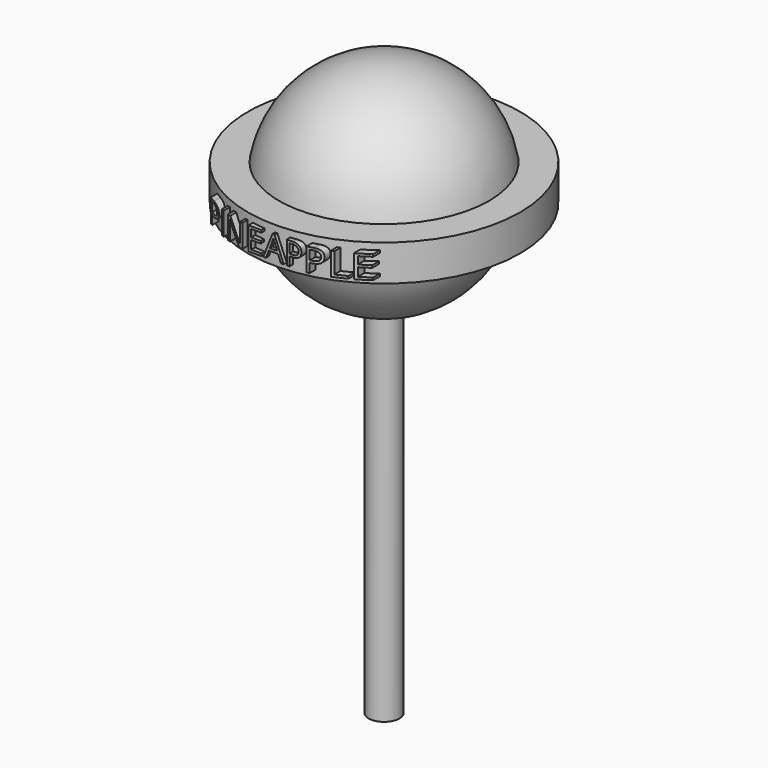
from build123d import *

# Parameters (mm, degrees)
F0_W         = 0.8679474239
F0_H         = 7.7723114803
F0_W_2       = 7.6306914445
F2_TEXT_SIZE = 6.9138606907
F3_DEPTH     = 30


# Not quite as in the source:
# - Text() gives the source's letters only with a copy of the font that has no kerning and outlines rounded to 1/6400 em; it was checked with that copy


with BuildPart() as f1:
    # F0 (on Front) → F1 (revolve)
    with BuildSketch(Plane.XZ):
        with BuildLine():
            Line((0, -18.649796024), (0, -22.9185808741))
            ThreePointArc((0, -22.9185808741), (1.6568504998, -22.8586131623), (3.305030521, -22.6790238445))
            Line((3.305030521, -22.6790238445), (3.305030521, -18.649796024))
            Line((3.305030521, -18.649796024), (0, -18.649796024))
        make_face()
        with BuildLine():
            ThreePointArc((3.305030521, -22.6790238445), (1.6568504998, -22.8586131623), (0, -22.9185808741))
            Line((0, -22.9185808741), (0, -100.3312021494))
            Line((0, -100.3312021494), (3.305030521, -100.3312021494))
            Line((3.305030521, -100.3312021494), (3.305030521, -22.6790238445))
        make_face()
        with BuildLine():
            Line((3.305030521, -18.649796024), (3.305030521, -22.6790238445))
            ThreePointArc((3.305030521, -22.6790238445), (15.9965132556, -16.4125839814), (22.5867027883, -3.8861557401))
            Line((22.5867027883, -3.8861557401), (0, -3.8861557401))
            Line((0, -3.8861557401), (0, -18.649796024))
            Line((0, -18.649796024), (3.305030521, -18.649796024))
        make_face()
        with BuildLine():
            Line((0, -3.8861557401), (22.5867027883, -3.8861557401))
            ThreePointArc((22.5867027883, -3.8861557401), (22.9185808741, 0), (22.5867027883, 3.8861557401))
            Line((22.5867027883, 3.8861557401), (0, 3.8861557401))
            Line((0, 3.8861557401), (0, -3.8861557401))
        make_face()
        with BuildLine():
            ThreePointArc((22.5867027883, 3.8861557401), (22.9185808741, 0), (22.5867027883, -3.8861557401))
            Line((22.5867027883, -3.8861557401), (29.2731001973, -3.8861557401))
            Line((29.2731001973, -3.8861557401), (29.2731001973, 3.8861557401))
            Line((29.2731001973, 3.8861557401), (22.5867027883, 3.8861557401))
        make_face()
        with Locations((-0.4339737119, 0)):
            Rectangle(F0_W, F0_H)
        with BuildLine():
            Line((0, 3.8861557401), (22.5867027883, 3.8861557401))
            ThreePointArc((22.5867027883, 3.8861557401), (14.7681443429, 17.5260737746), (0, 22.9185808741))
            Line((0, 22.9185808741), (0, 3.8861557401))
        make_face()
        with Locations((-4.6832931461, 0)):
            Rectangle(F0_W_2, F0_H)
    revolve(axis=Axis((0, 0, 27.5025516748), (0, 0, 1)))

    # F2 (on Front) → F3 (join)
    with BuildSketch(Plane.XZ):
        with Locations((-17.096086638, -2.4872907379)):
            Text('PINEAPPLE', F2_TEXT_SIZE, font='Open Sans', text_align=(TextAlign.LEFT, TextAlign.BOTTOM))
    extrude(amount=F3_DEPTH)

    # F4 (on Front) → F5 (revolve, cut)
    with BuildSketch(Plane.XZ):
        Polygon((30.7731001973, 5.3861557401), (30.7731001973, -5.3861557401), (23.5098041594, -5.3861557401), (27.8633013368, -23.0711500496), (47.6717241108, -19.9148624539), (53.548950702, 5.6619465016), (48.4335906804, 19.7643197477), (18.6121184379, 19.7643197477), (23.400966078, 5.3861557401), align=None)
    revolve(axis=Axis((0, 0, 32.1523994207), (0, 0, 1)), mode=Mode.SUBTRACT)


solid = f1.part
